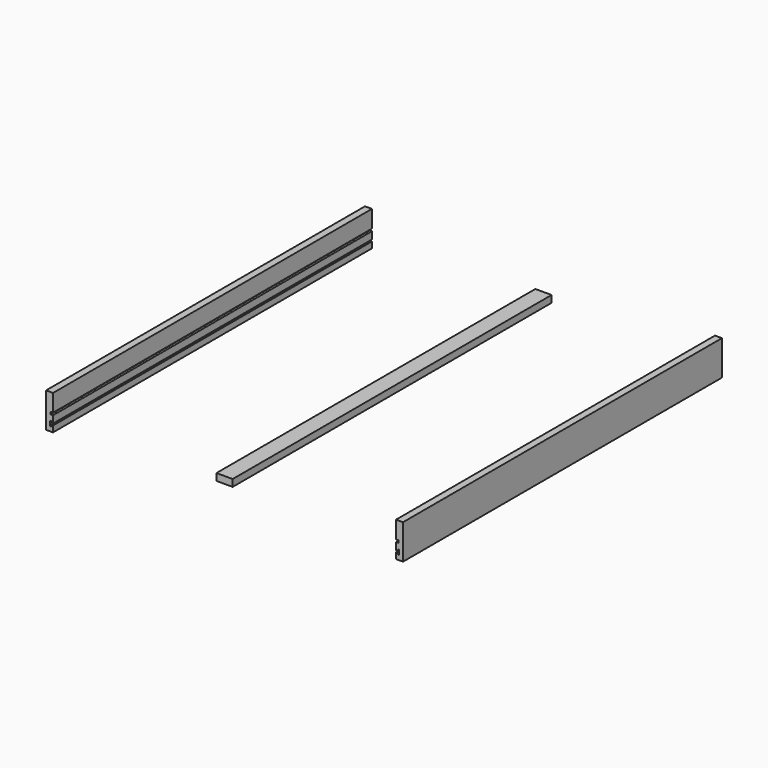
from build123d import *

# Parameters (mm, degrees)
F0_W     = 38.1
F0_H     = 190.5
F1_DEPTH = 1092.2
F0_W_2   = 88.9
F0_H_2   = 38.1
F2_W     = 12.7
F2_H     = 12.7
F3_DEPTH = 1092.2


# Not quite as in the source:
# - a feature names something its author has since deleted; it is built from what else it names


with BuildPart() as f1:
    # F0 (on Front) → F1 (new body, symmetric)
    with BuildSketch(Plane.XZ):
        with Locations((-958.85, 0)):
            Rectangle(F0_W, F0_H)
    extrude(amount=F1_DEPTH, both=True)


with BuildPart() as f1b:
    # F0 (on Front) → F1, piece 2 (new body, symmetric)
    with BuildSketch(Plane.XZ):
        with Locations((958.85, 0)):
            Rectangle(F0_W, F0_H)
    extrude(amount=F1_DEPTH, both=True)


with BuildPart() as f1c:
    # F0 (on Front) → F1, piece 3 (new body, symmetric)
    with BuildSketch(Plane.XZ):
        with Locations((0, -19.05)):
            Rectangle(F0_W_2, F0_H_2)
    extrude(amount=F1_DEPTH, both=True)


with BuildPart() as f3_tool:
    # F2 (on Front) → F3 (new body, symmetric)
    with BuildSketch(Plane.XZ):
        Polygon((-949.325, -61.9125), (-939.8, -61.9125), (-939.8, -57.15), (-955.675, -57.15), (-955.675, -69.85), (-949.325, -69.85), align=None)
        Polygon((-955.675, -57.15), (-939.8, -57.15), (-939.8, -52.3875), (-949.325, -52.3875), (-949.325, -44.45), (-955.675, -44.45), align=None)
        Polygon((949.325, -52.3875), (939.8, -52.3875), (939.8, -57.15), (955.675, -57.15), (955.675, -44.45), (949.325, -44.45), align=None)
        Polygon((955.675, -57.15), (939.8, -57.15), (939.8, -61.9125), (949.325, -61.9125), (949.325, -69.85), (955.675, -69.85), align=None)
        with Locations((-946.1499856949, -6.35)):
            Rectangle(F2_W, F2_H)
        with Locations((946.1499856949, -6.35)):
            Rectangle(F2_W, F2_H)
    extrude(amount=F3_DEPTH, both=True)


with BuildPart() as f1_1:
    add(f1.part)

    # F3: cut by f3_tool
    add(f3_tool.part, mode=Mode.SUBTRACT)


with BuildPart() as f1b_1:
    add(f1b.part)

    # F3: cut by f3_tool
    add(f3_tool.part, mode=Mode.SUBTRACT)


solid = Compound([f1c.part, f1_1.part, f1b_1.part])
